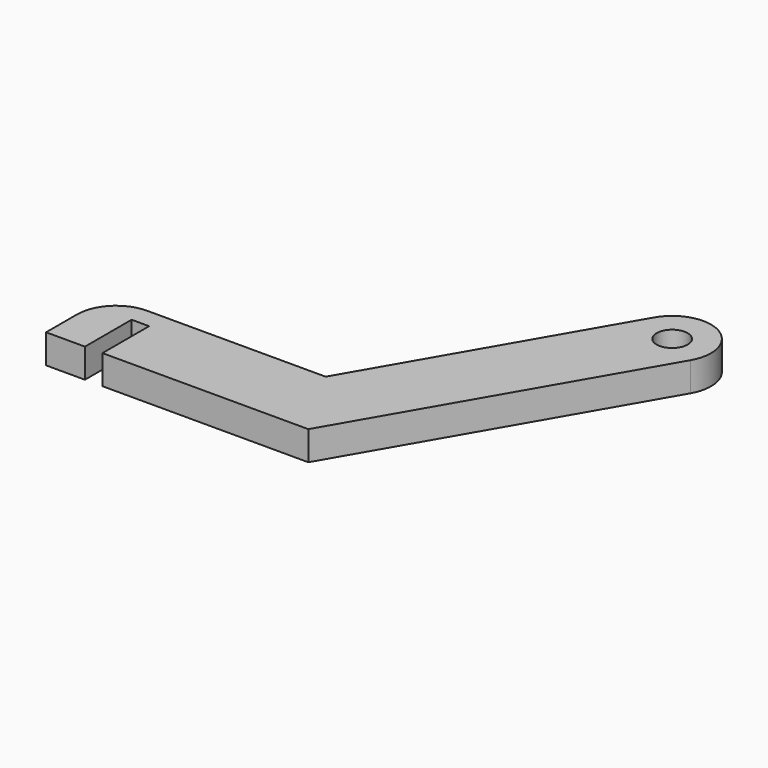
from build123d import *

# Parameters (mm, degrees)
F0_R     = 7.9957240037
F1_DEPTH = 15


# Not quite as in the source:
# - a feature names something its author has since deleted; it is built from what else it names


with BuildPart() as f1:
    # F0 (on Top) → F1 (new body)
    with BuildSketch(Plane.XY):
        with BuildLine():
            Line((60.2735915523, 0), (-31.5768626855, 0))
            ThreePointArc((-31.5768626855, 0), (-45.7189983092, -5.8578643763), (-51.5768626855, -20))
            Line((-51.5768626855, -20), (-51.5768626855, -40))
            Line((-51.5768626855, -40), (-31.5768626855, -40))
            Line((-31.5768626855, -40), (-31.5768626855, -10))
            Line((-31.5768626855, -10), (-22.5768626855, -10))
            Line((-22.5768626855, -10), (-22.5768626855, -40))
            Line((-22.5768626855, -40), (83.3676023199, -40))
            Line((83.3676023199, -40), (83.3676023199, -20))
            Line((83.3676023199, -20), (83.3676023199, 0))
            Line((83.3676023199, 0), (60.2735915523, 0))
        make_face()
        with BuildLine():
            Line((131.1026292389, 122.6794919243), (60.2735915523, 0))
            Line((60.2735915523, 0), (83.3676023199, 0))
            Line((83.3676023199, 0), (83.3676023199, -20))
            Line((83.3676023199, -20), (83.3676023199, -40))
            Line((83.3676023199, -40), (165.7436453902, 102.6794919243))
            ThreePointArc((165.7436453902, 102.6794919243), (167.7416538403, 117.8558728264), (158.4231373145, 130))
            ThreePointArc((158.4231373145, 130), (143.2467564125, 131.9980084501), (131.1026292389, 122.6794919243))
        make_face()
        with Locations((148.4231373145, 112.6794919243)):
            Circle(F0_R, mode=Mode.SUBTRACT)
    extrude(amount=F1_DEPTH)


solid = f1.part
